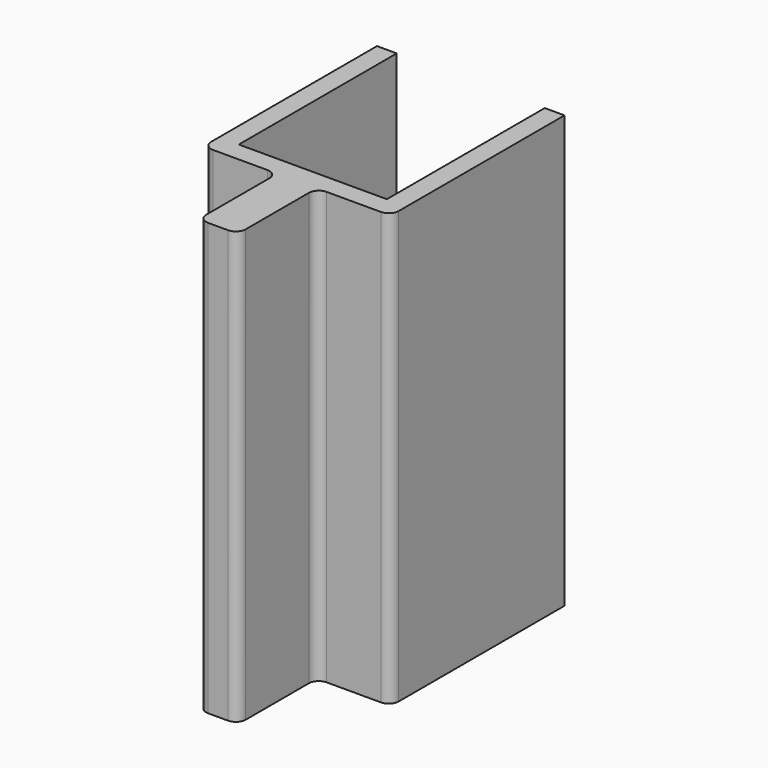
from build123d import *

# Parameters (mm, degrees)
F0_W     = 3.2
F0_H     = 8
F1_DEPTH = 35
F2_R     = 0.8


# Not quite as in the source:
# - a feature names something its author has since deleted; it is built from what else it names


with BuildPart() as f1:
    # F0 (on Top) → F1 (new body)
    with BuildSketch(Plane.XY):
        Polygon((0, 16), (0, 0), (-12, 0), (-12, 16), (-13.6, 16), (-13.6, -1.6), (-7.6, -1.6), (-4.4, -1.6), (1.6, -1.6), (1.6, 16), align=None)
        with Locations((-6, -5.6)):
            Rectangle(F0_W, F0_H)
    extrude(amount=F1_DEPTH)

    # F2
    f2_edges = [f1.edges().sort_by_distance(p)[0] for p in [
        (1.6, -1.6, 17.5),
        (-13.6, -1.6, 17.5),
        (-7.6, -1.6, 17.5),
        (-4.4, -1.6, 17.5),
        (-7.6, -9.6, 17.5),
        (-4.4, -9.6, 17.5),
    ]]
    fillet(f2_edges, radius=F2_R)


solid = f1.part
